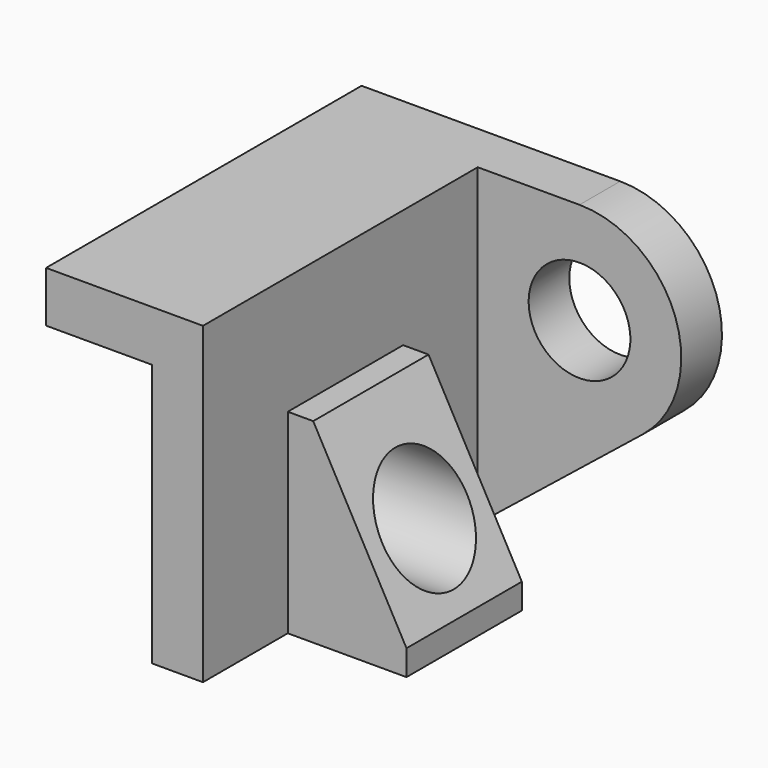
from build123d import *

# Parameters (mm, degrees)
F1_DEPTH  = 55
F2_W      = 34
F2_H      = 46
F3_DEPTH  = 28
F5_DEPTH  = 34
F6_R      = 12.5
F8_DEPTH  = 100
F10_DEPTH = 17
F11_W     = 12
F11_H     = 74
F12_DEPTH = 24
F14_DEPTH = 12
F15_DEPTH = 12
F16_R     = 12
F17_DEPTH = 25


# Not quite as in the source:
# - a feature of the source that left no trace in its solid (it failed there, or was rolled back) is left out


with BuildPart() as f1:
    # F0 (on Front) → F1 (new body, symmetric)
    with BuildSketch(Plane.XZ):
        Polygon((-3.9005428076, 30.4901414615), (-40.9005428076, 30.4901414615), (-40.9005428076, 18.4901414615), (-15.9005428076, 18.4901414615), (-15.9005428076, -43.5098585385), (-3.9005428076, -43.5098585385), align=None)
    extrude(amount=F1_DEPTH, both=True)

    # F2 (on face) → F3 (join)
    with BuildSketch(Plane.YZ.offset(-3.9005428076)):
        with Locations((-13, -20.5098585385)):
            Rectangle(F2_W, F2_H)
    extrude(amount=F3_DEPTH)

    # F4 (on face) → F5 (cut)
    with BuildSketch(Plane.XZ.offset(30)):
        Polygon((24.0994571924, 2.4901414615), (2.0994571924, 2.4901414615), (24.0994571924, -37.5098585385), align=None)
    extrude(amount=-F5_DEPTH, mode=Mode.SUBTRACT)

    # F6 (on face) → F8 (cut)
    with BuildSketch(Plane(origin=(-15.9005428076, 0, 0), x_dir=(0, -1, 0), z_dir=(-1, 0, 0))):
        with Locations((13, -20.5098585385)):
            Circle(F6_R)
    extrude(amount=-F8_DEPTH, mode=Mode.SUBTRACT)

    # F10 (cut): a face of the model
    f10_faces = [f1.faces().sort_by_distance(p)[0] for p in [
        (-14.5722599793, 55, 1.3184242898),
    ]]
    extrude(f10_faces, amount=-F10_DEPTH, mode=Mode.SUBTRACT)

    # F11 (on face) → F12 (join)
    with BuildSketch(Plane.YZ.offset(-3.9005428076)):
        with Locations((32, -6.5098585385)):
            Rectangle(F11_W, F11_H)
    extrude(amount=F12_DEPTH)

    # F13 (on face) → F14 (cut)
    with BuildSketch(Plane(origin=(0, 38, 0), x_dir=(-1, 0, 0), z_dir=(0, 1, 0))):
        with BuildLine():
            ThreePointArc((-20.0994571924, -17.5098585385), (-28.0551210727, -16.1529018901), (-35.1111607034, -12.2354762238))
            Line((-35.1111607034, -12.2354762238), (-20.0994571924, -24.2698585385))
            Line((-20.0994571924, -24.2698585385), (-20.0994571924, -17.5098585385))
        make_face()
        Polygon((3.9005428076, -43.5098585385), (-20.0994571924, -24.2698585385), (-20.0994571924, -43.5098585385), align=None)
    extrude(amount=-F14_DEPTH, mode=Mode.SUBTRACT)

    # F13 (on face) → F15 (join)
    with BuildSketch(Plane(origin=(0, 38, 0), x_dir=(-1, 0, 0), z_dir=(0, 1, 0))):
        with BuildLine():
            ThreePointArc((-35.1111607034, -12.2354762238), (-9.7139115703, -15.1464119177), (3.9005428076, 6.4901414615))
            ThreePointArc((3.9005428076, 6.4901414615), (-3.1288944439, 23.46070421), (-20.0994571924, 30.4901414615))
            ThreePointArc((-20.0994571924, 30.4901414615), (-42.742500544, 14.4458053418), (-35.1111607034, -12.2354762238))
        make_face()
        with BuildLine():
            ThreePointArc((-20.0994571924, -17.5098585385), (-28.0551210727, -16.1529018901), (-35.1111607034, -12.2354762238))
            Line((-35.1111607034, -12.2354762238), (-20.0994571924, -24.2698585385))
            Line((-20.0994571924, -24.2698585385), (-20.0994571924, -17.5098585385))
        make_face()
    extrude(amount=-F15_DEPTH)

    # F16 (on face) → F17 (cut)
    with BuildSketch(Plane(origin=(0, 38, 0), x_dir=(-1, 0, 0), z_dir=(0, 1, 0))):
        with Locations((-20.0994571924, 6.4901414615)):
            Circle(F16_R)
    extrude(amount=-F17_DEPTH, mode=Mode.SUBTRACT)


solid = f1.part
